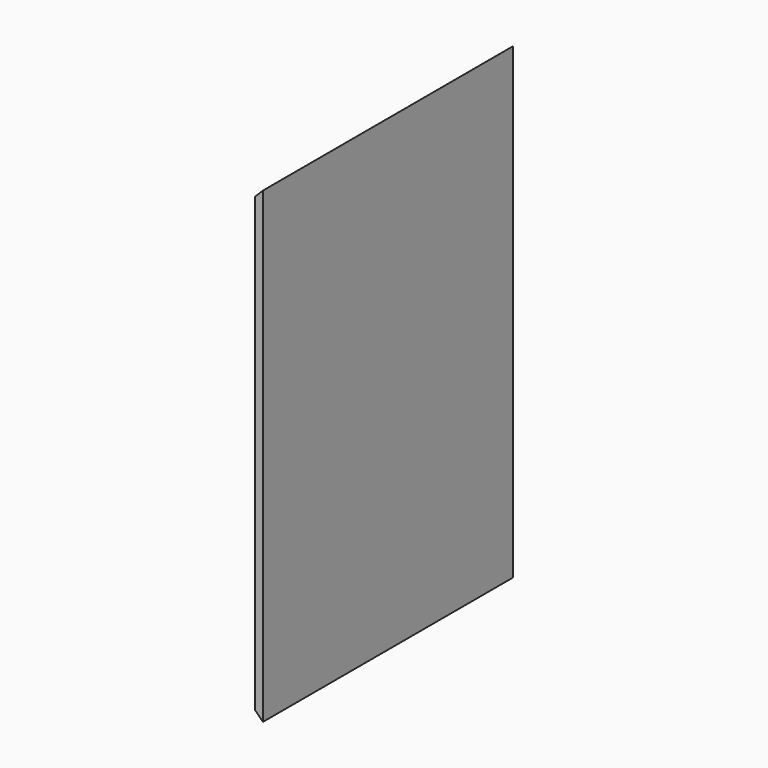
from build123d import *

# Parameters (mm, degrees)
F0_W     = 535
F0_H     = 800
F1_DEPTH = 14
F2_SIZE  = 13.99999


# Not quite as in the source:
# - a fillet or chamfer is up to 0.001 mm smaller than in the source, because OpenCascade refuses the exact size


with BuildPart() as f1:
    # F0 (on Right) → F1 (new body)
    with BuildSketch(Plane.YZ):
        Rectangle(F0_W, F0_H)
    extrude(amount=F1_DEPTH)

    # F2 (size 14 in the source; OpenCascade refuses exactly that, so slightly less here)
    f2_edges = [f1.edges().sort_by_distance(p)[0] for p in [
        (0, 0, 400),
        (0, 267.5, 0),
        (0, 0, -400),
    ]]
    chamfer(f2_edges, length=F2_SIZE)


solid = f1.part
